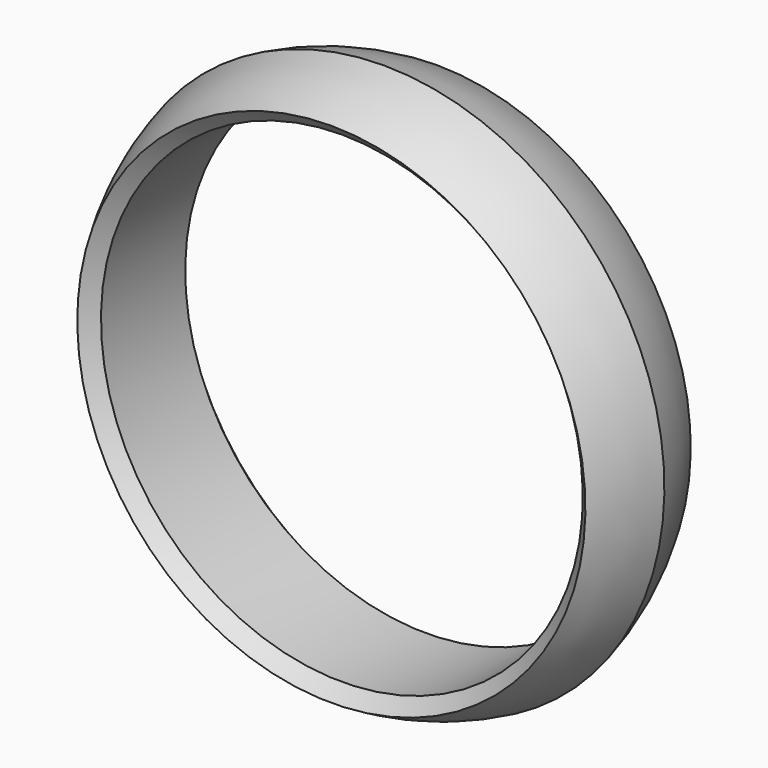
from build123d import *

# Parameters (mm, degrees)
F3_SIZE = 0.49999


# Not quite as in the source:
# - a fillet or chamfer is up to 0.001 mm smaller than in the source, because OpenCascade refuses the exact size


with BuildPart() as f2:
    # F1 (on Right) → F2 (revolve)
    with BuildSketch(Plane.YZ):
        with BuildLine():
            Line((-2.5, 9.1499136761), (0, 9.1499136761))
            Line((0, 9.1499136761), (2.5, 9.1499136761))
            Line((2.5, 9.1499136761), (2.5, 9.6499136761))
            ThreePointArc((2.5, 9.6499136761), (1.2898169642, 10.2494560866), (0, 10.6499136761))
            ThreePointArc((0, 10.6499136761), (-1.2898169642, 10.2494560866), (-2.5, 9.6499136761))
            Line((-2.5, 9.6499136761), (-2.5, 9.1499136761))
        make_face()
    revolve(axis=Axis((0, 0, 0), (0, -1, 0)))

    # F3 (size 0.5 in the source; OpenCascade refuses exactly that, so slightly less here)
    f3_edges = [f2.edges().sort_by_distance(p)[0] for p in [
        (0, -2.5, -9.149914),
        (0, 2.5, -9.149914),
    ]]
    chamfer(f3_edges, length=F3_SIZE)


solid = f2.part
